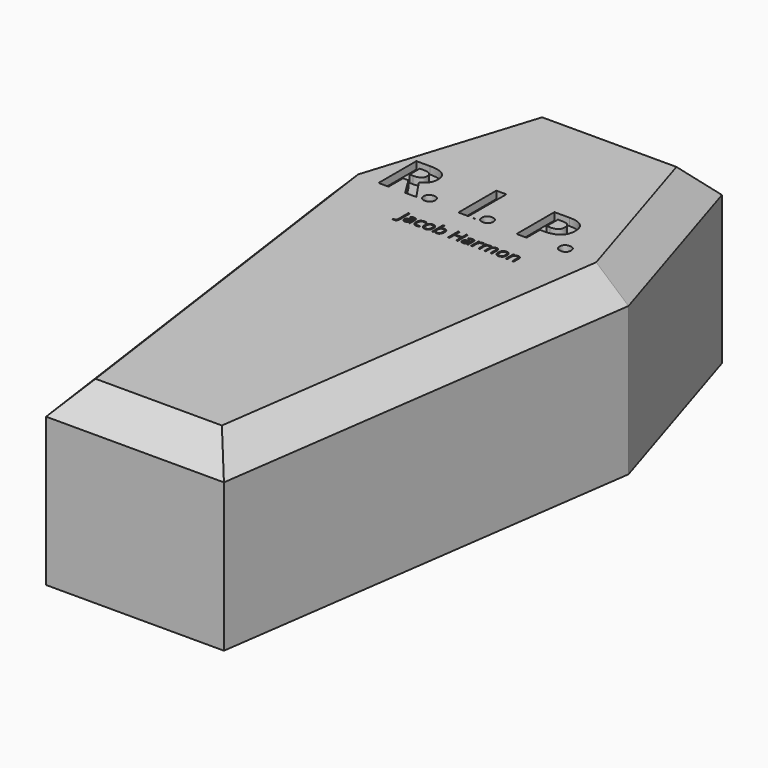
from build123d import *

# Parameters (mm, degrees)
F1_DEPTH       = 609.6
F2_SIZE        = 101.6
F3_TEXT_SIZE   = 227.3619174957
F3_TEXT_SIZE_2 = 1.7351499645
F3_TEXT_SIZE_3 = 61.3835536771
F4_DEPTH       = 25.4
F6_DEPTH       = 518.16


# Not quite as in the source:
# - Text() gives the source's letters only with a copy of the font that has no kerning and outlines rounded to 1/6400 em; it was checked with that copy


with BuildPart() as f1:
    # F0 (on Top) → F1 (new body)
    with BuildSketch(Plane.XY):
        Polygon((0, 1066.8), (-304.8, 1066.8), (-511.6426907063, 407.9234284878), (-304.8, -1066.8), (0, -1066.8), align=None)
        Polygon((304.8, 1066.8), (0, 1066.8), (0, -1066.8), (304.8, -1066.8), (511.6426907063, 407.9234284878), align=None)
    extrude(amount=F1_DEPTH)

    # F2
    f2_edges = [f1.edges().sort_by_distance(p)[0] for p in [
        (-408.221345, -329.438286, 609.6),
        (-408.221345, 737.361714, 609.6),
        (0, 1066.8, 609.6),
        (408.221345, 737.361714, 609.6),
        (408.221345, -329.438286, 609.6),
        (0, -1066.8, 609.6),
    ]]
    chamfer(f2_edges, length=F2_SIZE)

    # F3 (on face) → F4 (cut)
    with BuildSketch(Plane.XY.offset(609.6)):
        with Locations((-354.8097237945, 394.3114876747)):
            Text('R. I. P.', F3_TEXT_SIZE, font='Open Sans', font_style=FontStyle.BOLD, text_align=(TextAlign.LEFT, TextAlign.BOTTOM))
        with Locations((-11.6057132078, 393.0621797003)):
            Text('Jacob Harmon', F3_TEXT_SIZE_2, font='Open Sans', text_align=(TextAlign.LEFT, TextAlign.BOTTOM))
        with Locations((-168.5638576746, 264.2144858837)):
            Text('Jacob Harmon', F3_TEXT_SIZE_3, font='Open Sans', text_align=(TextAlign.LEFT, TextAlign.BOTTOM))
    extrude(amount=-F4_DEPTH, mode=Mode.SUBTRACT)

    # F5 (on face) → F6 (cut)
    with BuildSketch(Plane(origin=(0, 0, 0), x_dir=(1, 0, 0), z_dir=(0, 0, -1))):
        Polygon((-269.3681440078, -1018.5399899079), (269.3681440078, -1018.5399899079), (462.3390465338, -403.8506033801), (262.8364877031, 1018.5399899079), (-262.8364877031, 1018.5399899079), (-462.3390465338, -403.8506033801), align=None)
    extrude(amount=-F6_DEPTH, mode=Mode.SUBTRACT)


solid = f1.part
